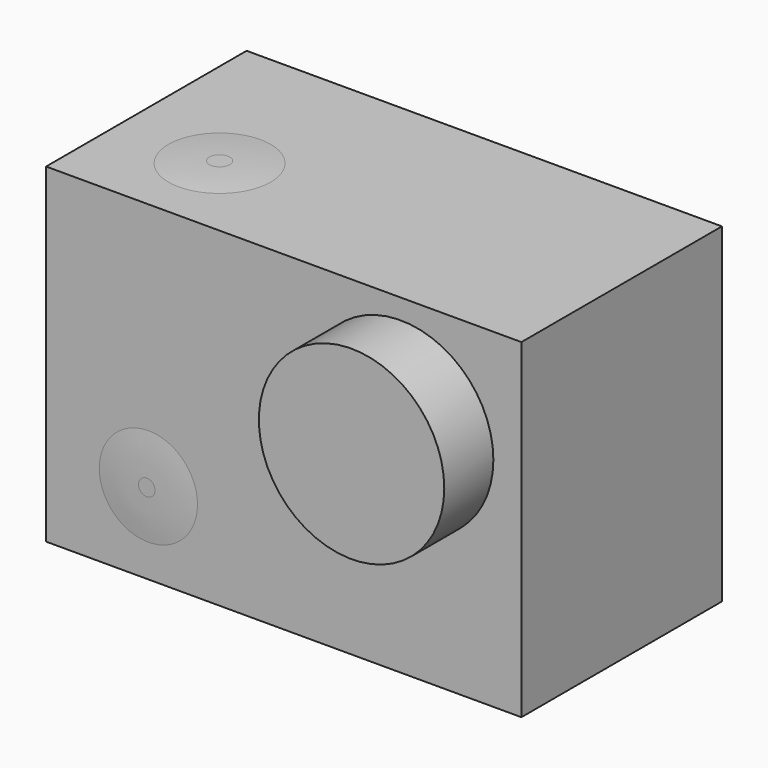
from build123d import *

# Parameters (mm, degrees)
F0_W      = 59.0042
F0_H      = 40.9956
F1_DEPTH  = 31.115
F3_R      = 11.5062
F4_DEPTH  = 7.62
F6_R      = 6.096
F7_DEPTH  = 0.254
F11_DEPTH = 0.254


# Not quite as in the source:
# - a fillet or chamfer that OpenCascade refuses, or shapes differently, is made with other operations: its cross-section is extruded or revolved along the edge and cut away or added


with BuildPart() as f1:
    # F0 (on Front) → F1 (new body)
    with BuildSketch(Plane.XZ):
        with Locations((-20.9379990903, -18.0528488383)):
            Rectangle(F0_W, F0_H)
    extrude(amount=F1_DEPTH)

    # F3 (on face) → F4 (join)
    with BuildSketch(Plane.XZ.offset(31.115)):
        with Locations((-6.4218990903, -11.5504488383)):
            Circle(F3_R)
    extrude(amount=F4_DEPTH)

    # F6 (on face) → F7 (join)
    with BuildSketch(Plane.XZ.offset(31.115)):
        with Locations((-37.7400990903, -28.3906488383)):
            Circle(F6_R)
    extrude(amount=F7_DEPTH)

    # F8: fillet of radius 50.8 on 1 edges, made by hand

    # F8_s1 → F8_t2 (revolve, cut)
    with BuildSketch(Plane.XY.offset(-28.3906488383)):
        with BuildLine():
            ThreePointArc((-31.6440990903, -31.115), (-34.1777451166, -31.3054602628), (-36.7177451166, -31.369))
            Line((-36.7177451166, -31.369), (-31.6440990903, -31.369))
            Line((-31.6440990903, -31.369), (-31.6440990903, -31.115))
        make_face()
    revolve(axis=Axis((-37.7400990903, -31.369, -28.3906488383), (0, -1, 0)), mode=Mode.SUBTRACT)

    # F10 (on face) → F11 (join)
    with BuildSketch(Plane.XY.offset(2.4449511617)):
        with BuildLine():
            ThreePointArc((-37.7400990903, -26.416), (-33.2499710298, -24.5561280605), (-31.3900990903, -20.066))
            ThreePointArc((-31.3900990903, -20.066), (-42.2302271509, -15.5758719395), (-37.7400990903, -26.416))
        make_face()
    extrude(amount=F11_DEPTH)

    # F12: fillet of radius 50.8 on 1 edges, made by hand

    # F12_s1 → F12_t2 (revolve, cut)
    with BuildSketch(Plane.YZ.offset(-37.7400990903)):
        with BuildLine():
            ThreePointArc((-26.416, 2.4449511617), (-23.8823539737, 2.6354114245), (-21.3423539737, 2.6989511617))
            Line((-21.3423539737, 2.6989511617), (-26.416, 2.6989511617))
            Line((-26.416, 2.6989511617), (-26.416, 2.4449511617))
        make_face()
    revolve(axis=Axis((-37.7400990903, -20.066, 2.6989511617), (0, 0, -1)), mode=Mode.SUBTRACT)


solid = f1.part
